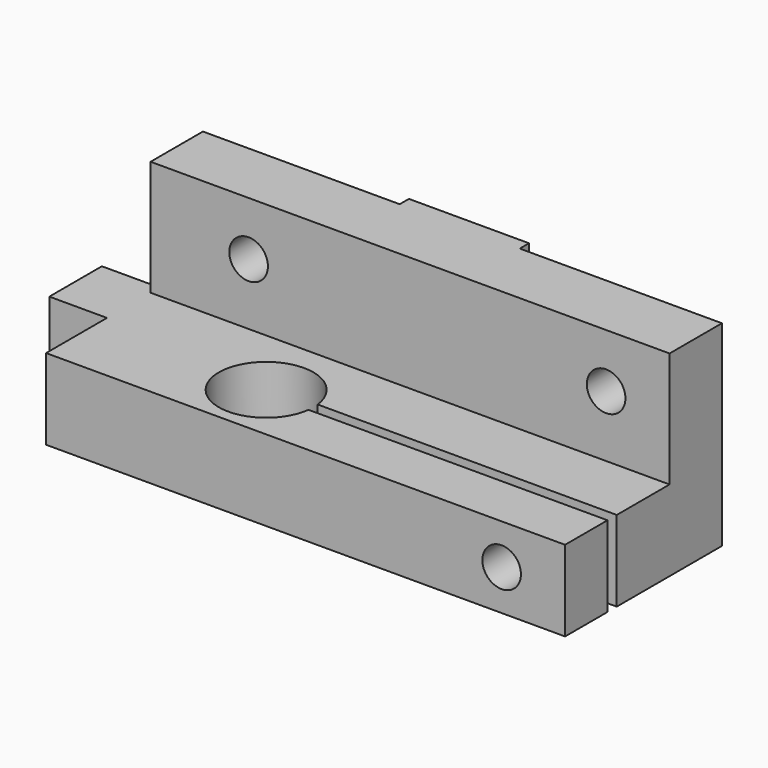
from build123d import *

# Parameters (mm, degrees)
F0_W          = 45
F0_H          = 17
F1_DEPTH      = 7
F4_DEPTH      = 25
F5_W          = 45
F5_H          = 5.6745335534
F6_DEPTH      = 10
F7_R          = 1.675
F8_DEPTH      = 25
F9_DEPTH      = 25
F10_TEXT_SIZE = 23.6111111111
F11_DEPTH     = 1
F12_W         = 5.7
F12_H         = 7
F13_DEPTH     = 5


# Not quite as in the source:
# - Text() gives the source's letters only with a copy of the font that has no kerning and outlines rounded to 1/6400 em; it was checked with that copy


with BuildPart() as f1:
    # F0 (on Top) → F1 (new body)
    with BuildSketch(Plane.XY):
        with Locations((22.5, 8.5)):
            Rectangle(F0_W, F0_H)
    extrude(amount=F1_DEPTH)

    # F3 (on face) → F4 (cut)
    with BuildSketch(Plane(origin=(0, 17, 0), x_dir=(-1, 0, 0), z_dir=(0, 1, 0))):
        with BuildLine():
            ThreePointArc((-41.175, 3.5), (-39.5, 1.825), (-37.825, 3.5))
            ThreePointArc((-37.825, 3.5), (-39.5, 5.175), (-41.175, 3.5))
        make_face()
    extrude(amount=-F4_DEPTH, mode=Mode.SUBTRACT)

    # F5 (on face) → F6 (join)
    with BuildSketch(Plane.XY.offset(7)):
        with Locations((22.5, 14.1627332233)):
            Rectangle(F5_W, F5_H)
    extrude(amount=F6_DEPTH)

    # F7 (on face) → F8 (cut)
    with BuildSketch(Plane(origin=(0, 17, 0), x_dir=(-1, 0, 0), z_dir=(0, 1, 0))):
        with Locations((-39.5, 12.325)):
            Circle(F7_R)
        with Locations((-8.5, 12.325)):
            Circle(F7_R)
    extrude(amount=-F8_DEPTH, mode=Mode.SUBTRACT)

    # F2 (on face) → F9 (cut)
    with BuildSketch(Plane.XY.offset(7)):
        with BuildLine():
            ThreePointArc((19.0693979899, 4.6), (19.0923423463, 4.8495321962), (19.1, 5.1))
            ThreePointArc((19.1, 5.1), (19.0923423463, 5.3504678038), (19.0693979899, 5.6))
            ThreePointArc((19.0693979899, 5.6), (10.9, 5.1), (19.0693979899, 4.6))
        make_face()
        with BuildLine():
            Line((45, 5.1), (19.1, 5.1))
            ThreePointArc((19.1, 5.1), (19.0923423463, 4.8495321962), (19.0693979899, 4.6))
            Line((19.0693979899, 4.6), (45, 4.6))
            Line((45, 4.6), (45, 5.1))
        make_face()
        with BuildLine():
            ThreePointArc((19.0693979899, 5.6), (19.0923423463, 5.3504678038), (19.1, 5.1))
            Line((19.1, 5.1), (45, 5.1))
            Line((45, 5.1), (45, 5.6))
            Line((45, 5.6), (19.0693979899, 5.6))
        make_face()
    extrude(amount=-F9_DEPTH, mode=Mode.SUBTRACT)

    # F10 (on face) → F11 (join)
    with BuildSketch(Plane(origin=(0, 17, 0), x_dir=(-1, 0, 0), z_dir=(0, 1, 0))):
        with Locations(Location((-14.9393391335, 17), (0, 0, -180))):
            Text('L', F10_TEXT_SIZE, font='Open Sans', font_style=FontStyle.BOLD, text_align=(TextAlign.LEFT, TextAlign.BOTTOM))
    extrude(amount=F11_DEPTH)

    # F12 (on face) → F13 (join)
    with BuildSketch(Plane(origin=(0, 0, 0), x_dir=(0, -1, 0), z_dir=(-1, 0, 0))):
        with Locations((-9.45, 3.5)):
            Rectangle(F12_W, F12_H)
    extrude(amount=F13_DEPTH)


solid = f1.part
